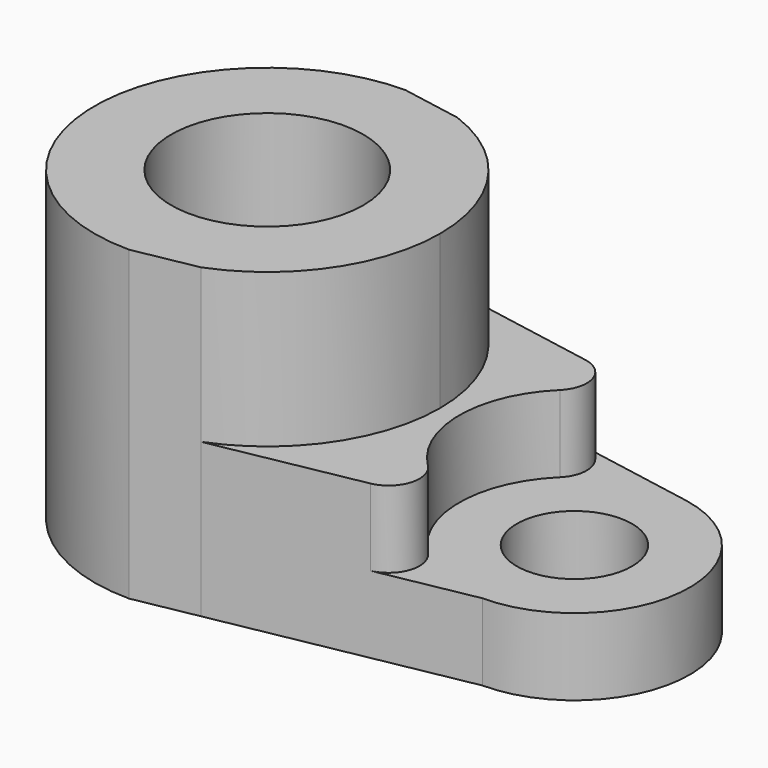
from build123d import *

# Parameters (mm, degrees)
F0_R        = 15.875
F0_R_2      = 9.525
F1_DEPTH    = 25.4
F2_DEPTH    = 25.4
F3_DEPTH    = 12.7
F4_T1_DEPTH = 53.6792843218
F4_T3_DEPTH = 61.8868884968


# Not quite as in the source:
# - a fillet or chamfer that OpenCascade refuses, or shapes differently, is made with other operations: its cross-section is extruded or revolved along the edge and cut away or added


with BuildPart() as f1:
    # F0 (on Top) → F1 (new body)
    with BuildSketch(Plane.XY):
        with BuildLine():
            Line((10.035773719, 26.7546981082), (0, 28.575))
            ThreePointArc((0, 28.575), (-28.575, 0), (0, -28.575))
            Line((0, -28.575), (10.3516981132, -26.6340566038))
            ThreePointArc((10.3516981132, -26.6340566038), (23.5831549902, -16.135842888), (28.575, 0))
            ThreePointArc((28.575, 0), (23.4872610048, 16.2751096921), (10.035773719, 26.7546981082))
        make_face()
        Circle(F0_R, mode=Mode.SUBTRACT)
        with BuildLine():
            Line((54.1998407335, 18.7441613039), (10.035773719, 26.7546981082))
            ThreePointArc((10.035773719, 26.7546981082), (23.4872610048, 16.2751096921), (28.575, 0))
            ThreePointArc((28.575, 0), (23.5831549902, -16.135842888), (10.3516981132, -26.6340566038))
            Line((10.3516981132, -26.6340566038), (50.8, -19.05))
            ThreePointArc((50.8, -19.05), (31.8266137334, 1.7067845735), (54.1998407335, 18.7441613039))
        make_face()
        with BuildLine():
            ThreePointArc((69.85, 0), (65.4230890371, 12.2093311452), (54.1998407335, 18.7441613039))
            ThreePointArc((54.1998407335, 18.7441613039), (31.8266137334, 1.7067845735), (50.8, -19.05))
            ThreePointArc((50.8, -19.05), (64.2703841816, -13.4703841816), (69.85, 0))
        make_face()
        with Locations((50.8, 0)):
            Circle(F0_R_2, mode=Mode.SUBTRACT)
    extrude(amount=-F1_DEPTH)

    # F0 (on Top) → F2 (join)
    with BuildSketch(Plane.XY):
        with BuildLine():
            Line((10.035773719, 26.7546981082), (0, 28.575))
            ThreePointArc((0, 28.575), (-28.575, 0), (0, -28.575))
            Line((0, -28.575), (10.3516981132, -26.6340566038))
            ThreePointArc((10.3516981132, -26.6340566038), (23.5831549902, -16.135842888), (28.575, 0))
            ThreePointArc((28.575, 0), (23.4872610048, 16.2751096921), (10.035773719, 26.7546981082))
        make_face()
        Circle(F0_R, mode=Mode.SUBTRACT)
    extrude(amount=F2_DEPTH)

    # F0 (on Top) → F3 (cut)
    with BuildSketch(Plane.XY):
        with BuildLine():
            ThreePointArc((69.85, 0), (65.4230890371, 12.2093311452), (54.1998407335, 18.7441613039))
            ThreePointArc((54.1998407335, 18.7441613039), (31.8266137334, 1.7067845735), (50.8, -19.05))
            ThreePointArc((50.8, -19.05), (64.2703841816, -13.4703841816), (69.85, 0))
        make_face()
        with Locations((50.8, 0)):
            Circle(F0_R_2, mode=Mode.SUBTRACT)
    extrude(amount=-F3_DEPTH, mode=Mode.SUBTRACT)

    # F4: fillet of radius 5.08 on 3 edges, made by hand

    # F4_s2 → F4_t1 (cut)
    with BuildSketch(Plane.XY.offset(-12.7)):
        with BuildLine():
            ThreePointArc((34.6890404798, -22.07080491), (38.6066005598, -18.5769977583), (37.3417274119, -13.4824848951))
            ThreePointArc((37.3417274119, -13.4824848951), (43.5177900762, -17.6031792193), (50.8, -19.05))
            Line((50.8, -19.05), (34.6890404798, -22.07080491))
        make_face()
    extrude(amount=F4_T1_DEPTH, mode=Mode.SUBTRACT)

    # F4_s4 → F4_t3 (cut)
    with BuildSketch(Plane.XY.offset(-12.7)):
        with BuildLine():
            ThreePointArc((34.8409541818, 22.2555017147), (38.7915508617, 18.7449449078), (37.4849973575, 13.6239937108))
            ThreePointArc((37.4849973575, 13.6239937108), (45.2204267219, 18.2145782832), (54.1998407335, 18.7441613039))
            Line((54.1998407335, 18.7441613039), (34.8409541818, 22.2555017147))
        make_face()
    extrude(amount=F4_T3_DEPTH, mode=Mode.SUBTRACT)


solid = f1.part
